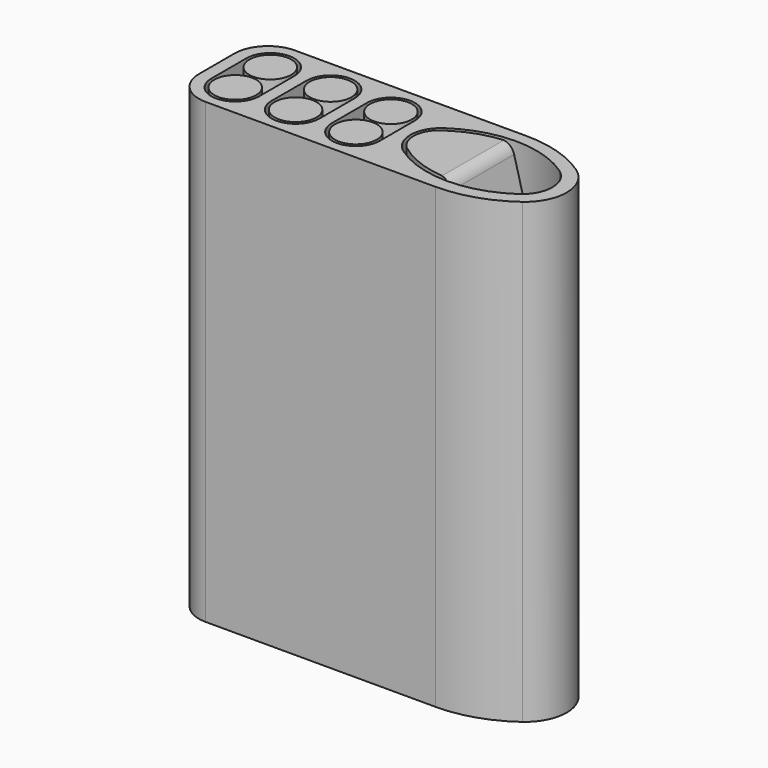
from build123d import *

# Parameters (mm, degrees)
F1_DEPTH = 2.286
F2_DEPTH = 82.55
F3_DEPTH = 82.55
F4_DEPTH = 82.55
F6_DEPTH = 12.7


with BuildPart() as f1:
    # F0 (on Top) → F1 (new body)
    with BuildSketch(Plane.XY):
        with BuildLine():
            ThreePointArc((-38.8948067667, 10.2486395534), (-43.3290625465, 8.3917710997), (-45.1170609992, 3.9293002248))
            Line((-45.1170609992, 3.9293002248), (-45.1170609992, -4.1909996693))
            ThreePointArc((-45.1170609992, -4.1909996693), (-43.2943864985, -8.5913251686), (-38.8940609992, -10.4139996693))
            Line((-38.8940609992, -10.4139996693), (3.7266951461, -10.4139996693))
            ThreePointArc((3.7266951461, -10.4139996693), (10.4351304739, -9.3421575585), (16.4756021904, -6.2333552972))
            ThreePointArc((16.4756021904, -6.2333552972), (19.6493908484, 0.1585761031), (16.2813302763, 6.4503079357))
            ThreePointArc((16.2813302763, 6.4503079357), (10.4640714266, 9.2771372612), (4.0697264362, 10.2486395534))
            Line((4.0697264362, 10.2486395534), (-38.8948067667, 10.2486395534))
        make_face()
        with BuildLine():
            Line((-33.9410609992, 3.9293002248), (-33.9410609992, -0.1308497222))
            Line((-33.9410609992, -0.1308497222), (-33.9410609992, -4.1909996693))
            ThreePointArc((-33.9410609992, -4.1909996693), (-38.3860609992, -8.6359996693), (-42.8310609992, -4.1909996693))
            Line((-42.8310609992, -4.1909996693), (-42.8310609992, 3.9293002248))
            ThreePointArc((-42.8310609992, 3.9293002248), (-38.3860609992, 8.3743002248), (-33.9410609992, 3.9293002248))
        make_face(mode=Mode.SUBTRACT)
        with BuildLine():
            Line((-22.7650609992, 3.9293002248), (-22.7650609992, -0.1308497222))
            Line((-22.7650609992, -0.1308497222), (-22.7650609992, -4.1909996693))
            ThreePointArc((-22.7650609992, -4.1909996693), (-27.2100609992, -8.6359996693), (-31.6550609992, -4.1909996693))
            Line((-31.6550609992, -4.1909996693), (-31.6550609992, -0.1308497222))
            Line((-31.6550609992, -0.1308497222), (-31.6550609992, 3.9293002248))
            ThreePointArc((-31.6550609992, 3.9293002248), (-27.2100609992, 8.3743002248), (-22.7650609992, 3.9293002248))
        make_face(mode=Mode.SUBTRACT)
        with BuildLine():
            ThreePointArc((-11.5890609992, -4.1909996693), (-16.0340609992, -8.6359996693), (-20.4790609992, -4.1909996693))
            Line((-20.4790609992, -4.1909996693), (-20.4790609992, -0.1308497222))
            Line((-20.4790609992, -0.1308497222), (-20.4790609992, 3.9293002248))
            ThreePointArc((-20.4790609992, 3.9293002248), (-16.0340609992, 8.3743002248), (-11.5890609992, 3.9293002248))
            Line((-11.5890609992, 3.9293002248), (-11.5890609992, -0.1380826775))
            Line((-11.5890609992, -0.1380826775), (-11.5890609992, -4.1909996693))
        make_face(mode=Mode.SUBTRACT)
        with BuildLine():
            ThreePointArc((-6.8362604978, -4.6544333602), (-8.6109304304, -2.6918958947), (-9.3030609992, -0.1380826775))
            ThreePointArc((-9.3030609992, -0.1380826775), (-8.6829118682, 2.6133376577), (-6.8149517752, 4.7265399425))
            ThreePointArc((-6.8149517752, 4.7265399425), (3.8387714228, 8.0331864612), (14.5025282944, 4.7590425175))
            ThreePointArc((14.5025282944, 4.7590425175), (16.9981004491, 0.0592448682), (14.5288463344, -4.6544333602))
            ThreePointArc((14.5288463344, -4.6544333602), (3.8462929183, -7.9611018574), (-6.8362604978, -4.6544333602))
        make_face(mode=Mode.SUBTRACT)
        with BuildLine():
            ThreePointArc((-6.8149517752, 4.7265399425), (-8.6829118682, 2.6133376577), (-9.3030609992, -0.1380826775))
            ThreePointArc((-9.3030609992, -0.1380826775), (-8.6109304304, -2.6918958947), (-6.8362604978, -4.6544333602))
            ThreePointArc((-6.8362604978, -4.6544333602), (3.8462929183, -7.9611018574), (14.5288463344, -4.6544333602))
            ThreePointArc((14.5288463344, -4.6544333602), (16.9981004491, 0.0592448682), (14.5025282944, 4.7590425175))
            ThreePointArc((14.5025282944, 4.7590425175), (3.8387714228, 8.0331864612), (-6.8149517752, 4.7265399425))
        make_face()
        with BuildLine():
            ThreePointArc((14.8385602726, -3.4910426491), (3.8316223107, -7.1990959272), (-7.1693058217, -3.4732507029))
            ThreePointArc((-7.1693058217, -3.4732507029), (-8.7275493844, -0.0546135102), (-7.3061653312, 3.4231545427))
            ThreePointArc((-7.3061653312, 3.4231545427), (3.2830324387, 7.2617905879), (14.0974344384, 4.1129899451))
            ThreePointArc((14.0974344384, 4.1129899451), (16.3951812505, 0.4988063216), (14.8385602726, -3.4910426491))
        make_face(mode=Mode.SUBTRACT)
        with BuildLine():
            ThreePointArc((-7.3061653312, 3.4231545427), (-8.7275493844, -0.0546135102), (-7.1693058217, -3.4732507029))
            ThreePointArc((-7.1693058217, -3.4732507029), (3.8316223107, -7.1990959272), (14.8385602726, -3.4910426491))
            ThreePointArc((14.8385602726, -3.4910426491), (16.3951812505, 0.4988063216), (14.0974344384, 4.1129899451))
            ThreePointArc((14.0974344384, 4.1129899451), (3.2830324387, 7.2617905879), (-7.3061653312, 3.4231545427))
        make_face()
        with BuildLine():
            Line((-33.9410609992, -4.1909996693), (-33.9410609992, -0.1308497222))
            Line((-33.9410609992, -0.1308497222), (-33.9410609992, 3.9293002248))
            ThreePointArc((-33.9410609992, 3.9293002248), (-38.3860609992, 8.3743002248), (-42.8310609992, 3.9293002248))
            Line((-42.8310609992, 3.9293002248), (-42.8310609992, -4.1909996693))
            ThreePointArc((-42.8310609992, -4.1909996693), (-38.3860609992, -8.6359996693), (-33.9410609992, -4.1909996693))
        make_face()
        with BuildLine():
            ThreePointArc((-34.5125609992, -4.1909996693), (-41.1250391161, -6.9299777862), (-38.3860609992, -0.3174996693))
            ThreePointArc((-38.3860609992, -0.3174996693), (-35.6470828822, -1.4520215523), (-34.5125609992, -4.1909996693))
        make_face(mode=Mode.SUBTRACT)
        with BuildLine():
            ThreePointArc((-34.5125609992, 3.9293002248), (-35.6470828822, 1.1903221079), (-38.3860609992, 0.0558002248))
            ThreePointArc((-38.3860609992, 0.0558002248), (-41.1250391161, 6.6682783418), (-34.5125609992, 3.9293002248))
        make_face(mode=Mode.SUBTRACT)
        with BuildLine():
            Line((-22.7650609992, -4.1909996693), (-22.7650609992, -0.1308497222))
            Line((-22.7650609992, -0.1308497222), (-22.7650609992, 3.9293002248))
            ThreePointArc((-22.7650609992, 3.9293002248), (-27.2100609992, 8.3743002248), (-31.6550609992, 3.9293002248))
            Line((-31.6550609992, 3.9293002248), (-31.6550609992, -0.1308497222))
            Line((-31.6550609992, -0.1308497222), (-31.6550609992, -4.1909996693))
            ThreePointArc((-31.6550609992, -4.1909996693), (-27.2100609992, -8.6359996693), (-22.7650609992, -4.1909996693))
        make_face()
        with BuildLine():
            ThreePointArc((-23.3365609992, -4.1909996693), (-29.9490391161, -6.9299777862), (-27.2100609992, -0.3174996693))
            ThreePointArc((-27.2100609992, -0.3174996693), (-24.4710828822, -1.4520215523), (-23.3365609992, -4.1909996693))
        make_face(mode=Mode.SUBTRACT)
        with BuildLine():
            ThreePointArc((-23.3365609992, 3.9293002248), (-24.4710828822, 1.1903221079), (-27.2100609992, 0.0558002248))
            ThreePointArc((-27.2100609992, 0.0558002248), (-29.9490391161, 6.6682783418), (-23.3365609992, 3.9293002248))
        make_face(mode=Mode.SUBTRACT)
        with BuildLine():
            Line((-20.4790609992, -0.1308497222), (-20.4790609992, -4.1909996693))
            ThreePointArc((-20.4790609992, -4.1909996693), (-16.0340609992, -8.6359996693), (-11.5890609992, -4.1909996693))
            Line((-11.5890609992, -4.1909996693), (-11.5890609992, -0.1380826775))
            Line((-11.5890609992, -0.1380826775), (-11.5890609992, 3.9293002248))
            ThreePointArc((-11.5890609992, 3.9293002248), (-16.0340609992, 8.3743002248), (-20.4790609992, 3.9293002248))
            Line((-20.4790609992, 3.9293002248), (-20.4790609992, -0.1308497222))
        make_face()
        with BuildLine():
            ThreePointArc((-12.1605609992, -4.1909996693), (-18.7730391161, -6.9299777862), (-16.0340609992, -0.3174996693))
            ThreePointArc((-16.0340609992, -0.3174996693), (-13.2950828822, -1.4520215523), (-12.1605609992, -4.1909996693))
        make_face(mode=Mode.SUBTRACT)
        with BuildLine():
            ThreePointArc((-12.1605609992, 3.9293002248), (-13.2950828822, 1.1903221079), (-16.0340609992, 0.0558002248))
            ThreePointArc((-16.0340609992, 0.0558002248), (-18.7730391161, 6.6682783418), (-12.1605609992, 3.9293002248))
        make_face(mode=Mode.SUBTRACT)
        with BuildLine():
            ThreePointArc((-34.5125609992, 3.9293002248), (-41.1250391161, 6.6682783418), (-38.3860609992, 0.0558002248))
            ThreePointArc((-38.3860609992, 0.0558002248), (-35.6470828822, 1.1903221079), (-34.5125609992, 3.9293002248))
        make_face()
        with BuildLine():
            ThreePointArc((-34.5125609992, -4.1909996693), (-35.6470828822, -1.4520215523), (-38.3860609992, -0.3174996693))
            ThreePointArc((-38.3860609992, -0.3174996693), (-41.1250391161, -6.9299777862), (-34.5125609992, -4.1909996693))
        make_face()
        with BuildLine():
            ThreePointArc((-23.3365609992, 3.9293002248), (-29.9490391161, 6.6682783418), (-27.2100609992, 0.0558002248))
            ThreePointArc((-27.2100609992, 0.0558002248), (-24.4710828822, 1.1903221079), (-23.3365609992, 3.9293002248))
        make_face()
        with BuildLine():
            ThreePointArc((-23.3365609992, -4.1909996693), (-24.4710828822, -1.4520215523), (-27.2100609992, -0.3174996693))
            ThreePointArc((-27.2100609992, -0.3174996693), (-29.9490391161, -6.9299777862), (-23.3365609992, -4.1909996693))
        make_face()
        with BuildLine():
            ThreePointArc((-12.1605609992, 3.9293002248), (-18.7730391161, 6.6682783418), (-16.0340609992, 0.0558002248))
            ThreePointArc((-16.0340609992, 0.0558002248), (-13.2950828822, 1.1903221079), (-12.1605609992, 3.9293002248))
        make_face()
        with BuildLine():
            ThreePointArc((-12.1605609992, -4.1909996693), (-13.2950828822, -1.4520215523), (-16.0340609992, -0.3174996693))
            ThreePointArc((-16.0340609992, -0.3174996693), (-18.7730391161, -6.9299777862), (-12.1605609992, -4.1909996693))
        make_face()
    extrude(amount=-F1_DEPTH)

    # F0 (on Top) → F4 (join)
    with BuildSketch(Plane.XY):
        with BuildLine():
            ThreePointArc((-38.8948067667, 10.2486395534), (-43.3290625465, 8.3917710997), (-45.1170609992, 3.9293002248))
            Line((-45.1170609992, 3.9293002248), (-45.1170609992, -4.1909996693))
            ThreePointArc((-45.1170609992, -4.1909996693), (-43.2943864985, -8.5913251686), (-38.8940609992, -10.4139996693))
            Line((-38.8940609992, -10.4139996693), (3.7266951461, -10.4139996693))
            ThreePointArc((3.7266951461, -10.4139996693), (10.4351304739, -9.3421575585), (16.4756021904, -6.2333552972))
            ThreePointArc((16.4756021904, -6.2333552972), (19.6493908484, 0.1585761031), (16.2813302763, 6.4503079357))
            ThreePointArc((16.2813302763, 6.4503079357), (10.4640714266, 9.2771372612), (4.0697264362, 10.2486395534))
            Line((4.0697264362, 10.2486395534), (-38.8948067667, 10.2486395534))
        make_face()
        with BuildLine():
            Line((-33.9410609992, 3.9293002248), (-33.9410609992, -0.1308497222))
            Line((-33.9410609992, -0.1308497222), (-33.9410609992, -4.1909996693))
            ThreePointArc((-33.9410609992, -4.1909996693), (-38.3860609992, -8.6359996693), (-42.8310609992, -4.1909996693))
            Line((-42.8310609992, -4.1909996693), (-42.8310609992, 3.9293002248))
            ThreePointArc((-42.8310609992, 3.9293002248), (-38.3860609992, 8.3743002248), (-33.9410609992, 3.9293002248))
        make_face(mode=Mode.SUBTRACT)
        with BuildLine():
            Line((-22.7650609992, 3.9293002248), (-22.7650609992, -0.1308497222))
            Line((-22.7650609992, -0.1308497222), (-22.7650609992, -4.1909996693))
            ThreePointArc((-22.7650609992, -4.1909996693), (-27.2100609992, -8.6359996693), (-31.6550609992, -4.1909996693))
            Line((-31.6550609992, -4.1909996693), (-31.6550609992, -0.1308497222))
            Line((-31.6550609992, -0.1308497222), (-31.6550609992, 3.9293002248))
            ThreePointArc((-31.6550609992, 3.9293002248), (-27.2100609992, 8.3743002248), (-22.7650609992, 3.9293002248))
        make_face(mode=Mode.SUBTRACT)
        with BuildLine():
            ThreePointArc((-11.5890609992, -4.1909996693), (-16.0340609992, -8.6359996693), (-20.4790609992, -4.1909996693))
            Line((-20.4790609992, -4.1909996693), (-20.4790609992, -0.1308497222))
            Line((-20.4790609992, -0.1308497222), (-20.4790609992, 3.9293002248))
            ThreePointArc((-20.4790609992, 3.9293002248), (-16.0340609992, 8.3743002248), (-11.5890609992, 3.9293002248))
            Line((-11.5890609992, 3.9293002248), (-11.5890609992, -0.1380826775))
            Line((-11.5890609992, -0.1380826775), (-11.5890609992, -4.1909996693))
        make_face(mode=Mode.SUBTRACT)
        with BuildLine():
            ThreePointArc((-6.8362604978, -4.6544333602), (-8.6109304304, -2.6918958947), (-9.3030609992, -0.1380826775))
            ThreePointArc((-9.3030609992, -0.1380826775), (-8.6829118682, 2.6133376577), (-6.8149517752, 4.7265399425))
            ThreePointArc((-6.8149517752, 4.7265399425), (3.8387714228, 8.0331864612), (14.5025282944, 4.7590425175))
            ThreePointArc((14.5025282944, 4.7590425175), (16.9981004491, 0.0592448682), (14.5288463344, -4.6544333602))
            ThreePointArc((14.5288463344, -4.6544333602), (3.8462929183, -7.9611018574), (-6.8362604978, -4.6544333602))
        make_face(mode=Mode.SUBTRACT)
    extrude(amount=F4_DEPTH)


with BuildPart() as f2:
    # F0 (on Top) → F2 (new body)
    with BuildSketch(Plane.XY):
        with BuildLine():
            ThreePointArc((-34.5125609992, 3.9293002248), (-41.1250391161, 6.6682783418), (-38.3860609992, 0.0558002248))
            ThreePointArc((-38.3860609992, 0.0558002248), (-35.6470828822, 1.1903221079), (-34.5125609992, 3.9293002248))
        make_face()
    extrude(amount=F2_DEPTH)


with BuildPart() as f2b:
    # F0 (on Top) → F2, piece 2 (new body)
    with BuildSketch(Plane.XY):
        with BuildLine():
            ThreePointArc((-34.5125609992, -4.1909996693), (-35.6470828822, -1.4520215523), (-38.3860609992, -0.3174996693))
            ThreePointArc((-38.3860609992, -0.3174996693), (-41.1250391161, -6.9299777862), (-34.5125609992, -4.1909996693))
        make_face()
    extrude(amount=F2_DEPTH)


with BuildPart() as f2c:
    # F0 (on Top) → F2, piece 3 (new body)
    with BuildSketch(Plane.XY):
        with BuildLine():
            ThreePointArc((-23.3365609992, 3.9293002248), (-29.9490391161, 6.6682783418), (-27.2100609992, 0.0558002248))
            ThreePointArc((-27.2100609992, 0.0558002248), (-24.4710828822, 1.1903221079), (-23.3365609992, 3.9293002248))
        make_face()
    extrude(amount=F2_DEPTH)


with BuildPart() as f2d:
    # F0 (on Top) → F2, piece 4 (new body)
    with BuildSketch(Plane.XY):
        with BuildLine():
            ThreePointArc((-23.3365609992, -4.1909996693), (-24.4710828822, -1.4520215523), (-27.2100609992, -0.3174996693))
            ThreePointArc((-27.2100609992, -0.3174996693), (-29.9490391161, -6.9299777862), (-23.3365609992, -4.1909996693))
        make_face()
    extrude(amount=F2_DEPTH)


with BuildPart() as f2e:
    # F0 (on Top) → F2, piece 5 (new body)
    with BuildSketch(Plane.XY):
        with BuildLine():
            ThreePointArc((-12.1605609992, 3.9293002248), (-18.7730391161, 6.6682783418), (-16.0340609992, 0.0558002248))
            ThreePointArc((-16.0340609992, 0.0558002248), (-13.2950828822, 1.1903221079), (-12.1605609992, 3.9293002248))
        make_face()
    extrude(amount=F2_DEPTH)


with BuildPart() as f2f:
    # F0 (on Top) → F2, piece 6 (new body)
    with BuildSketch(Plane.XY):
        with BuildLine():
            ThreePointArc((-12.1605609992, -4.1909996693), (-13.2950828822, -1.4520215523), (-16.0340609992, -0.3174996693))
            ThreePointArc((-16.0340609992, -0.3174996693), (-18.7730391161, -6.9299777862), (-12.1605609992, -4.1909996693))
        make_face()
    extrude(amount=F2_DEPTH)


with BuildPart() as f3:
    # F0 (on Top) → F3 (new body)
    with BuildSketch(Plane.XY):
        with BuildLine():
            ThreePointArc((-7.3061653312, 3.4231545427), (-8.7275493844, -0.0546135102), (-7.1693058217, -3.4732507029))
            ThreePointArc((-7.1693058217, -3.4732507029), (3.8316223107, -7.1990959272), (14.8385602726, -3.4910426491))
            ThreePointArc((14.8385602726, -3.4910426491), (16.3951812505, 0.4988063216), (14.0974344384, 4.1129899451))
            ThreePointArc((14.0974344384, 4.1129899451), (3.2830324387, 7.2617905879), (-7.3061653312, 3.4231545427))
        make_face()
    extrude(amount=F3_DEPTH)

    # F5 (on Front) → F6 (cut, symmetric)
    with BuildSketch(Plane.XZ):
        with BuildLine():
            Line((7.5214602545, 68.58), (16.4114602545, 68.58))
            Line((16.4114602545, 68.58), (19.0372634679, 68.58))
            Line((19.0372634679, 68.58), (19.0372634679, 88.6085554957))
            Line((19.0372634679, 88.6085554957), (16.4114602545, 88.6085554957))
            Line((16.4114602545, 88.6085554957), (-10.3636547431, 88.6085554957))
            Line((-10.3636547431, 88.6085554957), (-10.3636547431, 82.6238021255))
            Line((-10.3636547431, 82.6238021255), (1.6775887468, 82.6238021255))
            ThreePointArc((1.6775887468, 82.6238021255), (3.2136704438, 82.10668448), (4.1242915499, 80.7658911177))
            Line((4.1242915499, 80.7658911177), (7.5214602545, 68.58))
        make_face()
    extrude(amount=F6_DEPTH, both=True, mode=Mode.SUBTRACT)


with BuildPart() as f7_1:
    # F7: copy of F1
    add(f1.part)


solid = Compound([f1.part, f2.part, f2b.part, f2c.part, f2d.part, f2e.part, f2f.part, f3.part, f7_1.part])
